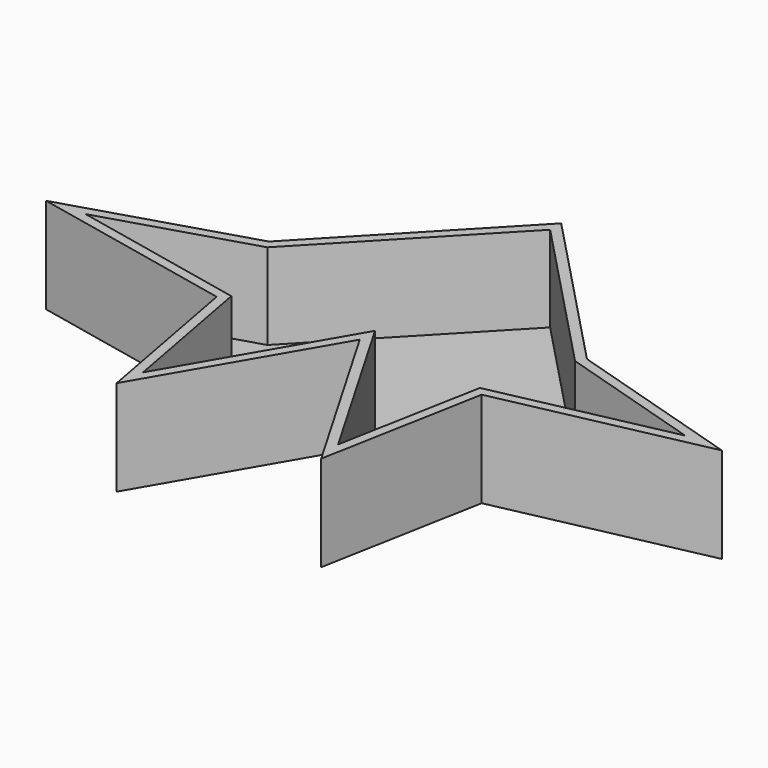
from build123d import *

# Parameters (mm, degrees)
F1_DEPTH = 10
F2_T     = -1


with BuildPart() as f1:
    # F0 (on Top) → F1 (new body)
    with BuildSketch(Plane.XY):
        Polygon((-46.061322093, 0), (-35.3632085025, 18.4245295823), (-24.6650949121, 0), (-21.4952845126, 17.037736252), (0, 21.5943418443), (-18.7216997147, 27.339624241), (-35.3632085025, 44.7735860944), (-52.0047172904, 27.339624241), (-70.7264170051, 21.5943418443), (-49.2311324924, 17.037736252), align=None)
    extrude(amount=F1_DEPTH)

    # F2
    f2_openings = [f1.faces().sort_by_distance(p)[0] for p in [
        (-35.363209, 22.945466, 10),
    ]]
    offset(amount=F2_T, openings=f2_openings, kind=Kind.INTERSECTION)


solid = f1.part
